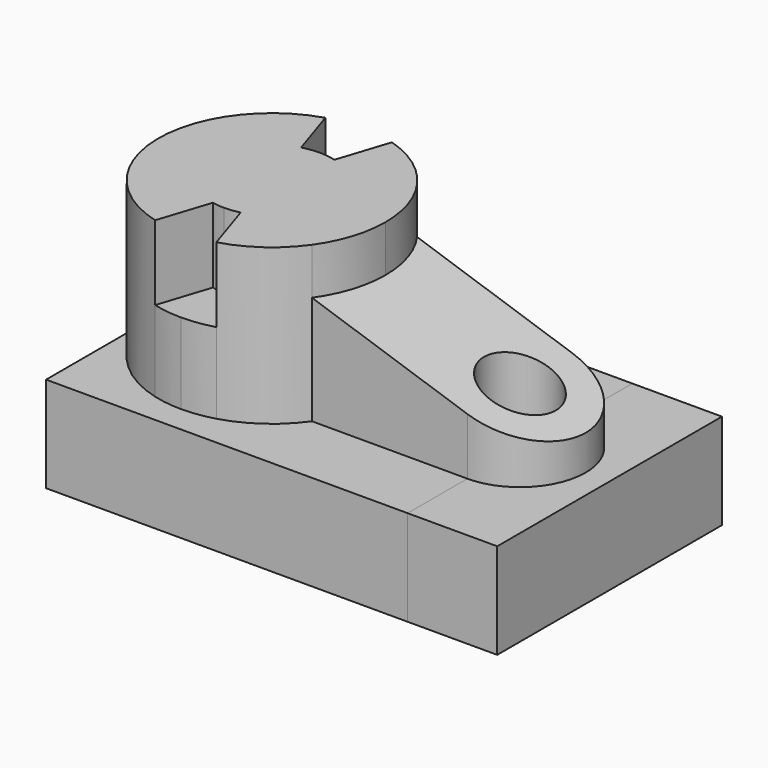
from build123d import *

# Parameters (mm, degrees)
F1_DEPTH = 52
F2_DEPTH = 27
F3_DEPTH = 32
F4_DEPTH = 32
F5_DEPTH = 12
F6_DEPTH = 24.4
F8_DEPTH = 74.5
F9_DEPTH = 32


with BuildPart() as f1:
    # F0 (on Top) → F1 (new body)
    with BuildSketch(Plane.XY):
        with BuildLine():
            ThreePointArc((-67.6857441339, 36.3163754823), (-87.0700692693, 22.5714612924), (-94.5, 1.882e-07))
            ThreePointArc((-94.5, 1.882e-07), (-86.6030709179, -23.1906257205), (-66.1944671175, -36.7425816636))
            Line((-66.1944671175, -36.7425816636), (-60.6154088174, -19.5720057803))
            ThreePointArc((-60.6154088174, -19.5720057803), (-76.4849090369, -0.7767952022), (-62.122189253, 19.1935142171))
            Line((-62.122189253, 19.1935142171), (-67.6857441339, 36.3163754823))
        make_face()
        with BuildLine():
            ThreePointArc((-18.5, 0), (-20.2964992214, 11.5458447667), (-25.5161332303, 22))
            ThreePointArc((-25.5161332303, 22), (-34.2843318109, 30.8295975795), (-45.4347623345, 36.3532737921))
            Line((-45.4347623345, 36.3532737921), (-50.9989145795, 19.2285740292))
            ThreePointArc((-50.9989145795, 19.2285740292), (-40.5309407226, 12.041143874), (-36.5, 0))
            ThreePointArc((-36.5, 0), (-40.6827641878, -12.2398958845), (-51.4815051263, -19.3601319521))
            Line((-51.4815051263, -19.3601319521), (-45.9138349552, -36.4956587781))
            ThreePointArc((-45.9138349552, -36.4956587781), (-34.4875508606, -30.9750235332), (-25.5161332303, -22))
            ThreePointArc((-25.5161332303, -22), (-20.2964992214, -11.5458447667), (-18.5, 0))
        make_face()
        with BuildLine():
            ThreePointArc((-36.5, 0), (-40.5309407226, 12.041143874), (-50.9989145795, 19.2285740292))
            ThreePointArc((-50.9989145795, 19.2285740292), (-53.7225443824, 19.8062045908), (-56.5, 20))
            Line((-56.5, 20), (-56.5, 0))
            Line((-56.5, 0), (-56.5, -20))
            ThreePointArc((-56.5, -20), (-53.9704386785, -19.8393880833), (-51.4815051263, -19.3601319521))
            ThreePointArc((-51.4815051263, -19.3601319521), (-40.6827641878, -12.2398958845), (-36.5, 0))
        make_face()
        with BuildLine():
            ThreePointArc((-56.5, 20), (-59.339869333, 19.797351898), (-62.122189253, 19.1935142171))
            ThreePointArc((-62.122189253, 19.1935142171), (-76.4849090369, -0.7767952022), (-60.6154088174, -19.5720057803))
            ThreePointArc((-60.6154088174, -19.5720057803), (-58.5688021163, -19.8927136863), (-56.5, -20))
            Line((-56.5, -20), (-56.5, 0))
            Line((-56.5, 0), (-56.5, 20))
        make_face()
    extrude(amount=F1_DEPTH)

    # F0 (on Top) → F5 (join)
    with BuildSketch(Plane.XY):
        with BuildLine():
            Line((26.5, 12), (26.5, 22))
            Line((26.5, 22), (-25.5161332303, 22))
            ThreePointArc((-25.5161332303, 22), (-20.2964992214, 11.5458447667), (-18.5, 0))
            ThreePointArc((-18.5, 0), (-20.2964992214, -11.5458447667), (-25.5161332303, -22))
            Line((-25.5161332303, -22), (26.5, -22))
            Line((26.5, -22), (26.5, -12))
            ThreePointArc((26.5, -12), (14.5, 0), (26.5, 12))
        make_face()
        with BuildLine():
            ThreePointArc((26.5, -22), (48.5, 0), (26.5, 22))
            Line((26.5, 22), (26.5, 12))
            ThreePointArc((26.5, 12), (34.9852813742, 8.4852813742), (38.5, 0))
            ThreePointArc((38.5, 0), (34.9852813742, -8.4852813742), (26.5, -12))
            Line((26.5, -12), (26.5, -22))
        make_face()
    extrude(amount=F5_DEPTH)

    # F6 (add): a face of the model
    f6_faces = [f1.faces().sort_by_distance(p)[0] for p in [
        (8.8600631876, 0, 12),
    ]]
    extrude(f6_faces, amount=F6_DEPTH)

    # F7 (on face) → F8 (cut)
    with BuildSketch(Plane.XZ.offset(22)):
        Polygon((26.5, 19.0561972631), (26.5, 36.4), (-25.5161332303, 36.4), align=None)
        Polygon((48.5, 11.720710434), (48.5, 36.4), (26.5, 36.4), (26.5, 19.0561972631), align=None)
    extrude(amount=-F8_DEPTH, mode=Mode.SUBTRACT)


with BuildPart() as f2:
    # F0 (on Top) → F2 (new body)
    with BuildSketch(Plane.XY):
        with BuildLine():
            Line((-56.5, -20), (-56.5, -38))
            ThreePointArc((-56.5, -38), (-51.1537411943, -37.6220349899), (-45.9138349552, -36.4956587781))
            Line((-45.9138349552, -36.4956587781), (-51.4815051263, -19.3601319521))
            ThreePointArc((-51.4815051263, -19.3601319521), (-53.9704386785, -19.8393880833), (-56.5, -20))
        make_face()
        with BuildLine():
            Line((-60.6154088174, -19.5720057803), (-66.1944671175, -36.7425816636))
            ThreePointArc((-66.1944671175, -36.7425816636), (-61.3878367804, -37.6843342997), (-56.5, -38))
            Line((-56.5, -38), (-56.5, -20))
            ThreePointArc((-56.5, -20), (-58.5688021163, -19.8927136863), (-60.6154088174, -19.5720057803))
        make_face()
    extrude(amount=F2_DEPTH)


with BuildPart() as f2b:
    # F0 (on Top) → F2, piece 2 (new body)
    with BuildSketch(Plane.XY):
        with BuildLine():
            Line((-50.9989145795, 19.2285740292), (-45.4347623345, 36.3532737921))
            ThreePointArc((-45.4347623345, 36.3532737921), (-50.9064503265, 37.586063934), (-56.5, 38))
            Line((-56.5, 38), (-56.5, 20))
            ThreePointArc((-56.5, 20), (-53.7225443824, 19.8062045908), (-50.9989145795, 19.2285740292))
        make_face()
        with BuildLine():
            ThreePointArc((-56.5, 38), (-62.1558700336, 37.5767366088), (-67.6857441339, 36.3163754823))
            Line((-67.6857441339, 36.3163754823), (-62.122189253, 19.1935142171))
            ThreePointArc((-62.122189253, 19.1935142171), (-59.339869333, 19.797351898), (-56.5, 20))
            Line((-56.5, 20), (-56.5, 38))
        make_face()
    extrude(amount=F2_DEPTH)


with BuildPart() as f3:
    # F0 (on Top) → F3 (new body)
    with BuildSketch(Plane.XY):
        with BuildLine():
            Line((26.5, 47), (-56.5, 47))
            Line((-56.5, 47), (-94.5, 47))
            Line((-94.5, 47), (-94.5, 1.882e-07))
            ThreePointArc((-94.5, 1.882e-07), (-87.0700692693, 22.5714612924), (-67.6857441339, 36.3163754823))
            ThreePointArc((-67.6857441339, 36.3163754823), (-62.1558700336, 37.5767366088), (-56.5, 38))
            ThreePointArc((-56.5, 38), (-50.9064503265, 37.586063934), (-45.4347623345, 36.3532737921))
            ThreePointArc((-45.4347623345, 36.3532737921), (-34.2843318109, 30.8295975795), (-25.5161332303, 22))
            Line((-25.5161332303, 22), (26.5, 22))
            Line((26.5, 22), (26.5, 47))
        make_face()
    extrude(amount=-F3_DEPTH)


with BuildPart() as f3b:
    # F0 (on Top) → F3, piece 2 (new body)
    with BuildSketch(Plane.XY):
        with BuildLine():
            ThreePointArc((-66.1944671175, -36.7425816636), (-86.6030709179, -23.1906257205), (-94.5, 1.882e-07))
            Line((-94.5, 1.882e-07), (-94.5, -47))
            Line((-94.5, -47), (-56.5, -47))
            Line((-56.5, -47), (26.5, -47))
            Line((26.5, -47), (26.5, -22))
            Line((26.5, -22), (-25.5161332303, -22))
            ThreePointArc((-25.5161332303, -22), (-34.4875508606, -30.9750235332), (-45.9138349552, -36.4956587781))
            ThreePointArc((-45.9138349552, -36.4956587781), (-51.1537411943, -37.6220349899), (-56.5, -38))
            ThreePointArc((-56.5, -38), (-61.3878367804, -37.6843342997), (-66.1944671175, -36.7425816636))
        make_face()
    extrude(amount=-F3_DEPTH)


with BuildPart() as f4:
    # F0 (on Top) → F4 (new body)
    with BuildSketch(Plane.XY):
        with BuildLine():
            Line((56.5, 47), (26.5, 47))
            Line((26.5, 47), (26.5, 22))
            ThreePointArc((26.5, 22), (48.5, 0), (26.5, -22))
            Line((26.5, -22), (26.5, -47))
            Line((26.5, -47), (56.5, -47))
            Line((56.5, -47), (56.5, 47))
        make_face()
    extrude(amount=-F4_DEPTH)


with BuildPart() as f9:
    # F0 (on Top) → F9 (new body)
    with BuildSketch(Plane.XY):
        with BuildLine():
            ThreePointArc((26.5, -22), (48.5, 0), (26.5, 22))
            Line((26.5, 22), (26.5, 12))
            ThreePointArc((26.5, 12), (34.9852813742, 8.4852813742), (38.5, 0))
            ThreePointArc((38.5, 0), (34.9852813742, -8.4852813742), (26.5, -12))
            Line((26.5, -12), (26.5, -22))
        make_face()
        with BuildLine():
            Line((26.5, 12), (26.5, 22))
            Line((26.5, 22), (-25.5161332303, 22))
            ThreePointArc((-25.5161332303, 22), (-20.2964992214, 11.5458447667), (-18.5, 0))
            ThreePointArc((-18.5, 0), (-20.2964992214, -11.5458447667), (-25.5161332303, -22))
            Line((-25.5161332303, -22), (26.5, -22))
            Line((26.5, -22), (26.5, -12))
            ThreePointArc((26.5, -12), (14.5, 0), (26.5, 12))
        make_face()
        with BuildLine():
            ThreePointArc((-18.5, 0), (-20.2964992214, 11.5458447667), (-25.5161332303, 22))
            ThreePointArc((-25.5161332303, 22), (-34.2843318109, 30.8295975795), (-45.4347623345, 36.3532737921))
            Line((-45.4347623345, 36.3532737921), (-50.9989145795, 19.2285740292))
            ThreePointArc((-50.9989145795, 19.2285740292), (-40.5309407226, 12.041143874), (-36.5, 0))
            ThreePointArc((-36.5, 0), (-40.6827641878, -12.2398958845), (-51.4815051263, -19.3601319521))
            Line((-51.4815051263, -19.3601319521), (-45.9138349552, -36.4956587781))
            ThreePointArc((-45.9138349552, -36.4956587781), (-34.4875508606, -30.9750235332), (-25.5161332303, -22))
            ThreePointArc((-25.5161332303, -22), (-20.2964992214, -11.5458447667), (-18.5, 0))
        make_face()
        with BuildLine():
            Line((-50.9989145795, 19.2285740292), (-45.4347623345, 36.3532737921))
            ThreePointArc((-45.4347623345, 36.3532737921), (-50.9064503265, 37.586063934), (-56.5, 38))
            Line((-56.5, 38), (-56.5, 20))
            ThreePointArc((-56.5, 20), (-53.7225443824, 19.8062045908), (-50.9989145795, 19.2285740292))
        make_face()
        with BuildLine():
            ThreePointArc((-56.5, 38), (-62.1558700336, 37.5767366088), (-67.6857441339, 36.3163754823))
            Line((-67.6857441339, 36.3163754823), (-62.122189253, 19.1935142171))
            ThreePointArc((-62.122189253, 19.1935142171), (-59.339869333, 19.797351898), (-56.5, 20))
            Line((-56.5, 20), (-56.5, 38))
        make_face()
        with BuildLine():
            ThreePointArc((-67.6857441339, 36.3163754823), (-87.0700692693, 22.5714612924), (-94.5, 1.882e-07))
            ThreePointArc((-94.5, 1.882e-07), (-86.6030709179, -23.1906257205), (-66.1944671175, -36.7425816636))
            Line((-66.1944671175, -36.7425816636), (-60.6154088174, -19.5720057803))
            ThreePointArc((-60.6154088174, -19.5720057803), (-76.4849090369, -0.7767952022), (-62.122189253, 19.1935142171))
            Line((-62.122189253, 19.1935142171), (-67.6857441339, 36.3163754823))
        make_face()
        with BuildLine():
            Line((-56.5, -20), (-56.5, -38))
            ThreePointArc((-56.5, -38), (-51.1537411943, -37.6220349899), (-45.9138349552, -36.4956587781))
            Line((-45.9138349552, -36.4956587781), (-51.4815051263, -19.3601319521))
            ThreePointArc((-51.4815051263, -19.3601319521), (-53.9704386785, -19.8393880833), (-56.5, -20))
        make_face()
        with BuildLine():
            Line((-60.6154088174, -19.5720057803), (-66.1944671175, -36.7425816636))
            ThreePointArc((-66.1944671175, -36.7425816636), (-61.3878367804, -37.6843342997), (-56.5, -38))
            Line((-56.5, -38), (-56.5, -20))
            ThreePointArc((-56.5, -20), (-58.5688021163, -19.8927136863), (-60.6154088174, -19.5720057803))
        make_face()
    extrude(amount=-F9_DEPTH)


solid = Compound([f1.part, f2.part, f2b.part, f3.part, f3b.part, f4.part, f9.part])
